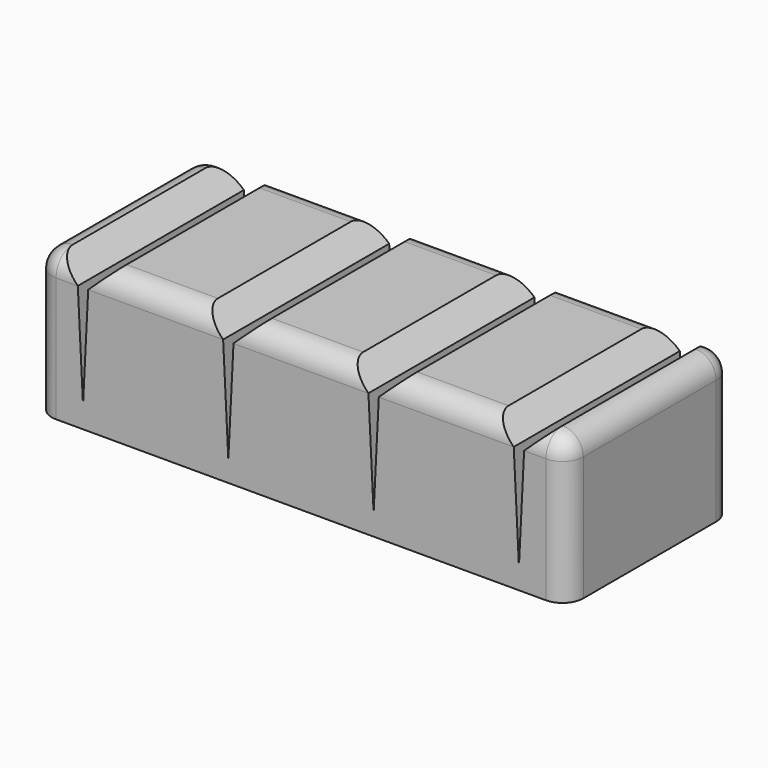
from build123d import *

# Parameters (mm, degrees)
F1_DEPTH = 50
F2_SIZE  = 5
F3_R     = 4.99999


# Not quite as in the source:
# - a fillet or chamfer is up to 0.001 mm smaller than in the source, because OpenCascade refuses the exact size


with BuildPart() as f1:
    # F0 (on Front) → F1 (new body)
    with BuildSketch(Plane.XZ):
        Polygon((-62.637026581, 14.7639395539), (-62.637026581, -20.2360604461), (65.362973419, -20.2360604461), (65.362973419, 14.7639395539), (55.362973419, 14.7639395539), (53.862973419, -15.2360604461), (52.362973419, 14.7639395539), (20.362973419, 14.7639395539), (18.862973419, -15.2360604461), (17.362973419, 14.7639395539), (-14.637026581, 14.7639395539), (-16.137026581, -15.2360604461), (-17.637026581, 14.7639395539), (-49.637026581, 14.7639395539), (-51.137026581, -15.2360604461), (-52.637026581, 14.7639395539), align=None)
    extrude(amount=F1_DEPTH)

    # F2
    f2_edges = [f1.edges().sort_by_distance(p)[0] for p in [
        (-52.637027, -25, 14.76394),
        (-49.637027, -25, 14.76394),
        (-17.637027, -25, 14.76394),
        (-14.637027, -25, 14.76394),
        (17.362973, -25, 14.76394),
        (20.362973, -25, 14.76394),
        (52.362973, -25, 14.76394),
        (55.362973, -25, 14.76394),
    ]]
    chamfer(f2_edges, length=F2_SIZE)

    # F3 (radius 5 in the source; OpenCascade refuses exactly that, so slightly less here)
    f3_edges = [f1.edges().sort_by_distance(p)[0] for p in [
        (-62.637027, -25, 14.76394),
        (-60.137027, -50, 14.76394),
        (-60.137027, 0, 14.76394),
        (-33.637027, -50, 14.76394),
        (-33.637027, 0, 14.76394),
        (1.362973, 0, 14.76394),
        (1.362973, -50, 14.76394),
        (36.362973, -50, 14.76394),
        (36.362973, 0, 14.76394),
        (62.862973, -50, 14.76394),
        (65.362973, -25, 14.76394),
        (62.862973, 0, 14.76394),
        (-62.637027, -50, -2.73606),
        (-62.637027, 0, -2.73606),
        (65.362973, -50, -2.73606),
        (65.362973, 0, -2.73606),
    ]]
    fillet(f3_edges, radius=F3_R)


solid = f1.part
